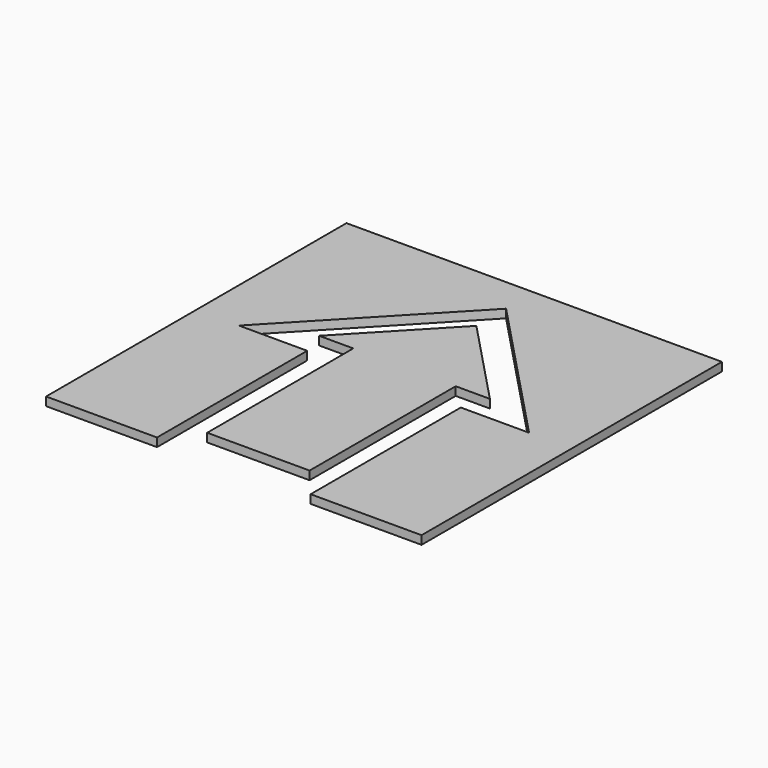
from build123d import *

# Parameters (mm, degrees)
F0_W     = 279.4
F0_H     = 279.4
F1_DEPTH = 6.35
F2_W     = 76.2
F2_H     = 12.7
F2_H_2   = 10.16
F3_DEPTH = 6.35


# Not quite as in the source:
# - a feature names something its author has since deleted; it is built from what else it names


with BuildPart() as f1:
    # F0 (on Top) → F1 (new body)
    with BuildSketch(Plane.XY):
        Rectangle(F0_W, F0_H)
    extrude(amount=F1_DEPTH)

    # F2 (on face) → F3 (cut)
    with BuildSketch(Plane.XY.offset(6.35)):
        Polygon((57.15, 0), (107.95, 0), (0, 113.5604063203), (-107.95, 0), (-57.15, 0), (-57.15, -139.7), (-38.1, -139.7), (-38.1, -127), (-38.1, -116.84), (-38.1, 0), (-38.1, 19.05), (-63.5574616586, 19.05), (0, 85.9106870833), (63.5574616586, 19.05), (38.1, 19.05), (38.1, 0), (38.1, -116.84), (38.1, -127), (38.1, -139.7), (57.15, -139.7), align=None)
        with Locations((0, -133.35)):
            Rectangle(F2_W, F2_H)
        with Locations((0, -121.92)):
            Rectangle(F2_W, F2_H_2)
    extrude(amount=-F3_DEPTH, mode=Mode.SUBTRACT)


solid = f1.part
